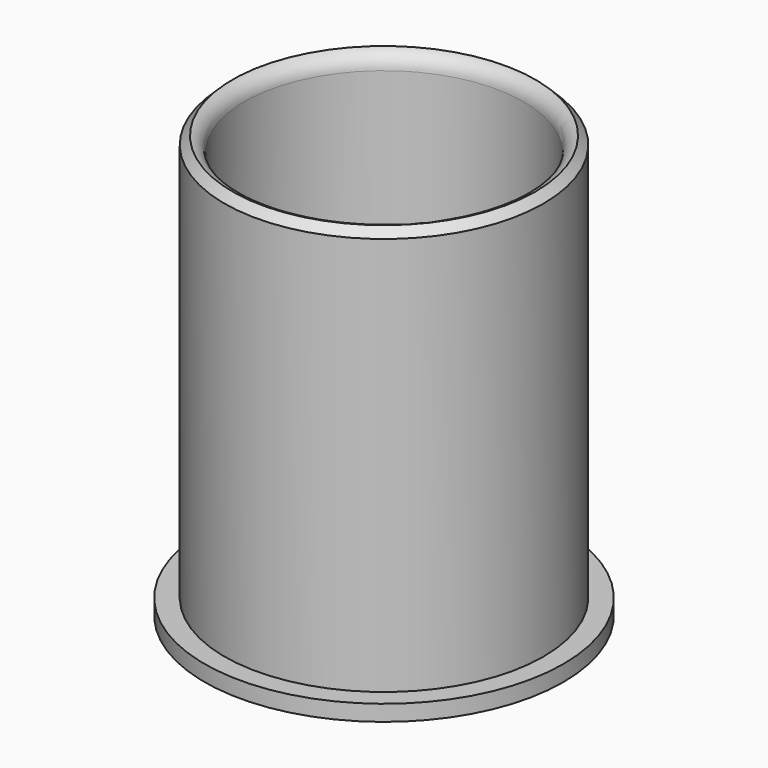
from build123d import *

# Parameters (mm, degrees)
F0_R     = 20
F1_DEPTH = 53
F0_R_2   = 22.5
F2_DEPTH = 2
F3_T     = -2.5
F4_DEPTH = 3
F5_SIZE  = 1
F7_R     = 2


# Not quite as in the source:
# - a fillet or chamfer that OpenCascade refuses, or shapes differently, is made with other operations: its cross-section is extruded or revolved along the edge and cut away or added


with BuildPart() as f1:
    # F0 (on Top) → F1 (new body)
    with BuildSketch(Plane.XY):
        Circle(F0_R)
    extrude(amount=F1_DEPTH)

    # F0 (on Top) → F2 (join)
    with BuildSketch(Plane.XY):
        Circle(F0_R_2)
        Circle(F0_R, mode=Mode.SUBTRACT)
    extrude(amount=F2_DEPTH)

    # F3
    f3_openings = [f1.faces().sort_by_distance(p)[0] for p in [
        (0, 0, 53),
    ]]
    offset(amount=F3_T, openings=f3_openings)

    # F4 (cut): a face of the model
    f4_faces = [f1.faces().sort_by_distance(p)[0] for p in [
        (0, 0, 2.5),
    ]]
    extrude(f4_faces, amount=-F4_DEPTH, mode=Mode.SUBTRACT)

    # F5
    f5_edges = [f1.edges().sort_by_distance(p)[0] for p in [
        (-20, 0, 53),
    ]]
    chamfer(f5_edges, length=F5_SIZE)

    # F6: fillet of radius 2 on 2 edges, made by hand

    # F6_s1 → F6_t2 (revolve, cut)
    with BuildSketch(Plane.XZ):
        with BuildLine():
            ThreePointArc((19, 53), (17.9188611699, 52.2882531983), (17.5, 51.0635083269))
            Line((17.5, 51.0635083269), (17.5, 53))
            Line((17.5, 53), (19, 53))
        make_face()
    revolve(axis=Axis((0, 0, 53), (0, 0, 1)), mode=Mode.SUBTRACT)

    # F7
    f7_edges = [f1.edges().sort_by_distance(p)[0] for p in [
        (-17.5, 0, 0),
    ]]
    fillet(f7_edges, radius=F7_R)


solid = f1.part
